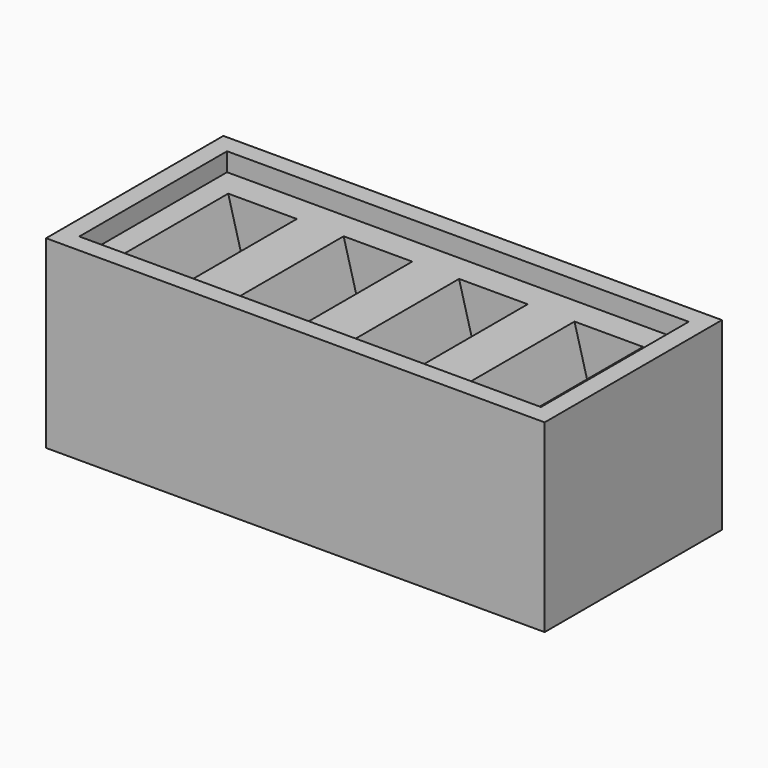
from build123d import *

# Parameters (mm, degrees)
F1_DEPTH = 50
F3_DEPTH = 9
F4_DEPTH = 9
F5_W     = 20
F5_H     = 2
F5_H_2   = 16
F6_DEPTH = 2
F8_DEPTH = 2


# Not quite as in the source:
# - a feature names something its author has since deleted; it is built from what else it names


with BuildPart() as f1:
    # F0 (on Right) → F1 (new body)
    with BuildSketch(Plane.YZ):
        Polygon((10, 18), (7, 18), (7, 6), (0, 6), (-7, 6), (-7, 18), (-10, 18), (-10, 20), (-12, 20), (-12, 0), (-10, 0), (-10, 16), (-9, 16), (-9, 4), (0, 4), (9, 4), (9, 16), (10, 16), (10, 0), (12, 0), (12, 20), (10, 20), align=None)
    extrude(amount=F1_DEPTH)

    # F2 (on Front) → F3 (join, symmetric)
    with BuildSketch(Plane.XZ):
        Polygon((37.4974226119, 16), (38.5692193817, 16), (41.7846096908, 4), (45.7128129211, 4), (48.9282032303, 16), (50, 16), (50, 18), (49.4641016151, 18), (47.4641016151, 18), (44.248711306, 6), (43.248711306, 6), (40.0333209968, 18), (38.0333209968, 18), (37.4974226119, 18), (36.9615242271, 18), (34.9615242271, 18), (31.7461339179, 6), (30.7461339179, 6), (27.5307436087, 18), (25.5307436087, 18), (24.9948452239, 18), (24.458946839, 18), (22.458946839, 18), (19.2435565298, 6), (18.2435565298, 6), (15.0281662206, 18), (13.0281662206, 18), (12.4922678358, 18), (11.9563694509, 18), (9.9563694509, 18), (6.7409791417, 6), (5.7409791417, 6), (2.5255888326, 18), (0.5255888326, 18), (-0.0103095523, 18), (-0.0103095523, 16), (1.0614872174, 16), (4.2768775266, 4), (8.2050807569, 4), (11.4204710661, 16), (12.4922678358, 16), (13.5640646055, 16), (16.7794549147, 4), (20.707658145, 4), (23.9230484541, 16), (24.9948452239, 16), (26.0666419936, 16), (29.2820323028, 4), (33.210235533, 4), (36.4256258422, 16), align=None)
    extrude(amount=F3_DEPTH, both=True)

    # F2 (on Front) → F4 (cut, symmetric)
    with BuildSketch(Plane.XZ):
        Polygon((48.9282032303, 16), (45.7128129211, 4), (50, 4), (50, 16), align=None)
        Polygon((41.7846096908, 4), (38.5692193817, 16), (37.4974226119, 16), (36.4256258422, 16), (33.210235533, 4), (37.4974226119, 4), align=None)
        Polygon((24.9948452239, 4), (29.2820323028, 4), (26.0666419936, 16), (24.9948452239, 16), (23.9230484541, 16), (20.707658145, 4), align=None)
        Polygon((12.4922678358, 4), (16.7794549147, 4), (13.5640646055, 16), (12.4922678358, 16), (11.4204710661, 16), (8.2050807569, 4), align=None)
        Polygon((-0.0103095523, 4), (4.2768775266, 4), (1.0614872174, 16), (-0.0103095523, 16), align=None)
    extrude(amount=F4_DEPTH, both=True, mode=Mode.SUBTRACT)

    # F5 (on face) → F6 (join)
    with BuildSketch(Plane.YZ.offset(50)):
        with Locations((0, 19)):
            Rectangle(F5_W, F5_H)
        Polygon((-10, 20), (-12, 20), (-12, 0), (-10, 0), (-10, 16), (10, 16), (10, 0), (12, 0), (12, 20), (10, 20), (10, 18), (-10, 18), align=None)
        with Locations((0, 8)):
            Rectangle(F5_W, F5_H_2)
    extrude(amount=F6_DEPTH)

    # F7 (on face) → F8 (join)
    with BuildSketch(Plane(origin=(0, 0, 0), x_dir=(0, -1, 0), z_dir=(-1, 0, 0))):
        Polygon((12, 20), (10, 20), (10, 18), (9, 18), (9, 16), (10, 16), (10, 0), (12, 0), align=None)
        Polygon((10, 20), (-12, 20), (-12, 0), (10, 0), (10, 16), (9, 16), (9, 18), (10, 18), align=None)
    extrude(amount=F8_DEPTH)


solid = f1.part
